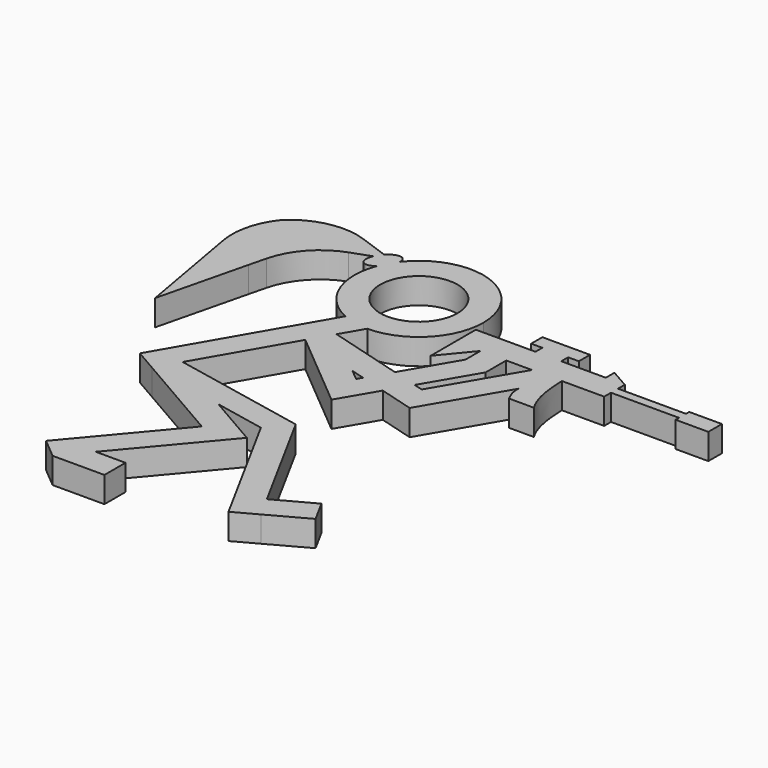
from build123d import *

# Parameters (mm, degrees)
F0_W        = 7.9140815362
F0_H        = 1.0166466236
F0_W_2      = 3
F0_H_2      = 1
F0_R        = 4.5
F1_DEPTH    = 3
F2_T1_DEPTH = 3
F2_T3_DEPTH = 28.8894591878
F2_T5_DEPTH = 23.3681675465


# Not quite as in the source:
# - a fillet or chamfer that OpenCascade refuses, or shapes differently, is made with other operations: its cross-section is extruded or revolved along the edge and cut away or added


with BuildPart() as f1:
    # F0 (on Top) → F1 (new body)
    with BuildSketch(Plane.XY):
        Polygon((13.4622063488, -0.5), (14.7628532723, -0.5), (17.7628532723, -0.5), (19.0106034279, -0.5), (19.0106034279, 1.1280798353), (13.4622063488, 1.1280798353), align=None)
        Polygon((10.7628532723, -6.6854998734), (7.292940495, -12.6047210891), (10.2724858996, -13.4541141028), (13.7628532723, -7.5), (13.7628532723, -4.5), (10.7628532723, -4.5), align=None)
        with BuildLine():
            Line((-14.7281754762, 1.7223088071), (-8.4750935815, 3.9539961383))
            add(Edge.make_bspline(
                [(-7.8951590451, 4.8302771503), (-8.2686696422, 4.4379188565), (-8.4750935815, 3.9539961383)],
                knots=[1.3532409109, 1.3532409109, 1.3532409109, 1.9420651459, 1.9420651459, 1.9420651459], degree=2, weights=[1, 0.9569728978, 1]))
            Line((-7.8951590451, 4.8302771503), (-16.1634236574, 7.7945101075))
            Line((-16.1634236574, 7.7945101075), (-21.7940099537, 1.9431159599))
            Line((-21.7940099537, 1.9431159599), (-18.813110888, -14.8382401094))
            Line((-18.813110888, -14.8382401094), (-16.2738263607, -4.4602961279))
            Line((-16.2738263607, -4.4602961279), (-14.7281754762, 1.7223088071))
        make_face()
        Polygon((-4.1330147038, -41.823990643), (-6.7042714065, -44.8882950559), (-0.673970324, -44.8882950559), (-0.673970324, -41.823990643), align=None)
        Polygon((7.292940495, -12.6047210891), (-1.5, -10.0980762114), (4.1472461263, -14.8274837274), (5.7260863187, -15.2775711223), align=None)
        Polygon((33.0707170069, -2.4889647029), (33.0707170069, -3.5056113265), (33.0707170069, -3.9974618703), (36.8696413934, -3.9974618703), (36.8696413934, -2.0199886058), (33.0707170069, -2.0199886058), align=None)
        Polygon((18.2495536771, -36.9809648262), (13.8269943134, -39.3890709971), (15.287962521, -42.0721830228), (19.7105218846, -39.6640768519), align=None)
        with Locations((29.1136762388, -2.9972880147)):
            Rectangle(F0_W, F0_H)
        Polygon((-9.0024047358, -23.0926223927), (-10.5024047358, -25.6906986041), (-1.2683224195, -27.5578969), align=None)
        with BuildLine():
            add(Edge.make_bspline(
                [(-8.4750935815, 3.9539961383), (-9.9447387818, 0.5086849859), (-7.0206677136, 2.6382238069)],
                knots=[1.9420651459, 1.9420651459, 1.9420651459, 4.2160777827, 4.2160777827, 4.2160777827], degree=2, weights=[1, 0.420312788, 1]))
            ThreePointArc((-7.0206677136, 2.6382238069), (-6.5359057109, 3.6785780593), (-5.8980778892, 4.6327828799))
            add(Edge.make_bspline(
                [(-5.8980778892, 4.6327828799), (-5.898901623, 5.1347150622), (-6.2072743134, 5.3597039059)],
                knots=[5.6018784444, 5.6018784444, 5.6018784444, 6.2831853072, 6.2831853072, 6.2831853072], degree=2, weights=[1, 0.9425365533, 1]))
            add(Edge.make_bspline(
                [(-6.2072743134, 5.3597039059), (-6.9059188983, 5.8694352869), (-7.8951590451, 4.8302771503)],
                knots=[0, 0, 0, 1.3532409109, 1.3532409109, 1.3532409109], degree=2, weights=[1, 0.7796933083, 1]))
            add(Edge.make_bspline(
                [(-7.8951590451, 4.8302771503), (-8.2686696422, 4.4379188565), (-8.4750935815, 3.9539961383)],
                knots=[1.3532409109, 1.3532409109, 1.3532409109, 1.9420651459, 1.9420651459, 1.9420651459], degree=2, weights=[1, 0.9569728978, 1]))
        make_face()
        Polygon((8.7628532723, -4.5), (10.7628532723, -4.5), (13.7628532723, -4.5), (16.7579661865, -4.5), (20.2354351463, -4.5), (25.1566354707, -4.5), (25.1566354707, -3.5056113265), (25.1566354707, -2.4889647029), (25.1566354707, -1.5), (22.9422256299, -1.5), (17.7628532723, -1.5), (14.7628532723, -1.5), (8.7628532723, -1.5), align=None)
        with BuildLine():
            Line((20.2354351463, -4.5), (18.0979731586, -8.1462329624))
            add(Edge.make_bspline(
                [(18.0979731586, -8.1462329624), (18.0473234504, -9.0044103563), (18.3297842741, -9.5410849899), (18.6251010746, -10.1915458217)],
                knots=[0, 0, 0, 0, 2.1121478481, 2.1121478481, 2.1121478481, 2.1121478481], degree=3))
            Line((18.6251010746, -10.1915458217), (21.5215887874, -10.1907448843))
            add(Edge.make_bspline(
                [(20.2354351463, -4.5), (20.3352533281, -6.2362966128), (20.3635003418, -8.2417670637), (21.5215887874, -10.1907448843)],
                knots=[0, 0, 0, 0, 5.8342753215, 5.8342753215, 5.8342753215, 5.8342753215], degree=3))
        make_face()
        with BuildLine():
            ThreePointArc((0, -7.5), (-1.5760318318, -7.3325386917), (-3.0816838363, -6.8376329774))
            Line((-3.0816838363, -6.8376329774), (-13.1004809472, -24.1906986041))
            Line((-13.1004809472, -24.1906986041), (-10.5024047358, -25.6906986041))
            Line((-10.5024047358, -25.6906986041), (-9.0024047358, -23.0926223927))
            Line((-9.0024047358, -23.0926223927), (-3.0228838472, -12.7357884087))
            Line((-3.0228838472, -12.7357884087), (-1.5, -10.0980762114))
            Line((-1.5, -10.0980762114), (0, -7.5))
        make_face()
        with BuildLine():
            ThreePointArc((-5.8980778892, 4.6327828799), (-6.5359057109, 3.6785780593), (-7.0206677136, 2.6382238069))
            add(Edge.make_bspline(
                [(-7.0206677136, 2.6382238069), (-5.896148589, 3.4571871888), (-5.8980778892, 4.6327828799)],
                knots=[4.2160777827, 4.2160777827, 4.2160777827, 5.6018784444, 5.6018784444, 5.6018784444], degree=2, weights=[1, 0.7693966053, 1]))
        make_face()
        Polygon((11.3319195864, -13.7561318437), (10.2724858996, -13.4541141028), (8.7056317233, -16.1269641361), (12.7446108147, -17.2783748907), (18.0979731586, -8.1462329624), (20.2354351463, -4.5), (16.7579661865, -4.5), align=None)
        Polygon((7.8259082511, -8.0615244806), (10.7628532723, -4.5), (8.7628532723, -4.5), (8.7628532723, -1.5), (7.8259082511, -1.5), align=None)
        with Locations((16.2628532723, -1)):
            Rectangle(F0_W_2, F0_H_2)
        with BuildLine():
            ThreePointArc((-7.0206677136, 2.6382238069), (-6.9254849764, -2.8788292484), (-3.0816838363, -6.8376329774))
            ThreePointArc((-3.0816838363, -6.8376329774), (-1.5760318318, -7.3325386917), (0, -7.5))
            ThreePointArc((0, -7.5), (5.3033008589, -5.3033008589), (7.5, 0))
            ThreePointArc((7.5, 0), (2.4509606107, 7.088215014), (-5.8980778892, 4.6327828799))
            add(Edge.make_bspline(
                [(-7.0206677136, 2.6382238069), (-5.896148589, 3.4571871888), (-5.8980778892, 4.6327828799)],
                knots=[4.2160777827, 4.2160777827, 4.2160777827, 5.6018784444, 5.6018784444, 5.6018784444], degree=2, weights=[1, 0.7693966053, 1]))
        make_face()
        Circle(F0_R, mode=Mode.SUBTRACT)
        Polygon((-1.2683224195, -27.5578969), (-10.5024047358, -25.6906986041), (0.2696389092, -31.9099409022), (-9.0024047358, -42.9599322269), (-6.7042714065, -44.8882950559), (-4.1330147038, -41.823990643), (4.8659055679, -31.0994950798), align=None)
        Polygon((10.2724858996, -13.4541141028), (7.292940495, -12.6047210891), (5.7260863187, -15.2775711223), (8.7056317233, -16.1269641361), align=None)
        Polygon((22.9422256299, -0.2355174292), (22.9422256299, -1.5), (25.1566354707, -1.5), align=None)
        Polygon((6.6801939907, -26.2637573918), (-9.0024047358, -23.0926223927), (-1.2683224195, -27.5578969), (4.616944438, -28.7479404659), (12.6532249158, -43.5068111111), (15.287962521, -42.0721830228), (13.8269943134, -39.3890709971), align=None)
        Polygon((4.1472461263, -14.8274837274), (-1.5, -10.0980762114), (-3.0228838472, -12.7357884087), (6.1770209488, -20.4404462041), (8.7056317233, -16.1269641361), (5.7260863187, -15.2775711223), (5.3831728236, -15.8625370756), align=None)
    extrude(amount=F1_DEPTH)

    # F2: fillet of radius 8 on 3 edges, made by hand

    # F2_s2 → F2_t1 (join)
    with BuildSketch(Plane.XY):
        with BuildLine():
            ThreePointArc((-15.7668598362, -2.4324295718), (-13.9323879929, 1.0007952454), (-10.6947478435, 3.1618148779))
            Line((-10.6947478435, 3.1618148779), (-14.7281754762, 1.7223088071))
            Line((-14.7281754762, 1.7223088071), (-15.7668598362, -2.4324295718))
        make_face()
    extrude(amount=F2_T1_DEPTH)

    # F2_s4 → F2_t3 (cut)
    with BuildSketch(Plane.XY.offset(-12.9447295939)):
        with BuildLine():
            ThreePointArc((-11.2892959012, 6.0470998817), (-15.8144489693, 6.3053971181), (-19.7536720515, 4.0634673109))
            Line((-19.7536720515, 4.0634673109), (-16.1634236574, 7.7945101075))
            Line((-16.1634236574, 7.7945101075), (-11.2892959012, 6.0470998817))
        make_face()
    extrude(amount=F2_T3_DEPTH, mode=Mode.SUBTRACT)

    # F2_s6 → F2_t5 (cut)
    with BuildSketch(Plane.XY.offset(-10.1840837733)):
        with BuildLine():
            ThreePointArc((-18.9694325729, 4.8784613548), (-20.8588428617, 1.6587603608), (-21.0815566526, -2.0677318634))
            Line((-21.0815566526, -2.0677318634), (-21.7940099537, 1.9431159599))
            Line((-21.7940099537, 1.9431159599), (-18.9694325729, 4.8784613548))
        make_face()
    extrude(amount=F2_T5_DEPTH, mode=Mode.SUBTRACT)


solid = f1.part
